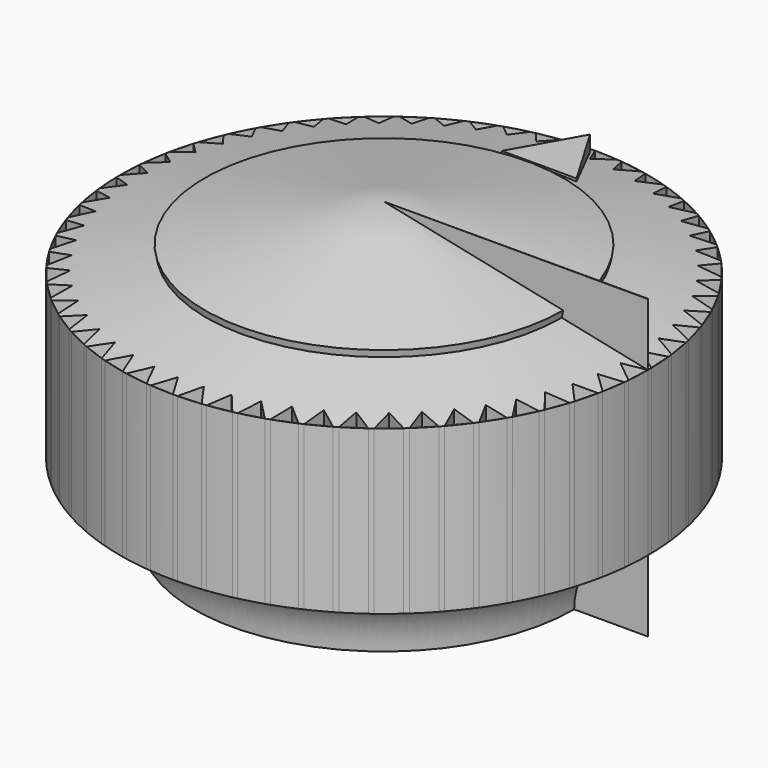
from build123d import *

# Parameters (mm, degrees)
F1_R             = 14.097
F2_DEPTH         = 15.875
F4_ANGLE         = 359.9
F6_DEPTH         = 0.635
F7_DEPTH         = 8.3566
F9_DEPTH         = 11.43
F11_DEPTH        = 15.876
F11_COPIES_COUNT = 60


# Not quite as in the source:
# - a pattern or mirror of a feature is missing from the dataset's text; its kind, count and spacing are read off the source's solid


with BuildPart() as f2:
    # F1 (on Top) → F2 (new body)
    with BuildSketch(Plane.XY):
        Circle(F1_R)
    extrude(amount=F2_DEPTH)

    # F3 (on Front) → F4 (revolve, cut)
    with BuildSketch(Plane.XZ):
        Polygon((14.5759196816, 15.875), (0, 15.875), (9.5739045491, 13.8729814857), (9.4959196816, 13.5000480326), (14.4887969726, 12.4559773794), (14.5759196816, 12.827), align=None)
        with BuildLine():
            Line((14.097, 0), (14.097, 3.8218105259))
            ThreePointArc((14.097, 3.8218105259), (11.3203081245, 2.7434560638), (10.16, 0))
            Line((10.16, 0), (14.097, 0))
        make_face()
    revolve(axis=Axis((0, 0, 15.875), (0, 0, -1)), revolution_arc=F4_ANGLE, mode=Mode.SUBTRACT)

    # F8 (on face) → F9 (cut)
    with BuildSketch(Plane(origin=(0, 0, 0), x_dir=(1, 0, 0), z_dir=(0, 0, -1))):
        with BuildLine():
            Line((-2.2079380086, -2.54), (2.2079380086, -2.54))
            ThreePointArc((2.2079380086, -2.54), (0, 3.3655), (-2.2079380086, -2.54))
        make_face()
    extrude(amount=-F9_DEPTH, mode=Mode.SUBTRACT)

    # F10 (on Top) → F11 (cut, through all)
    with BuildSketch(Plane.XY):
        Polygon((-14.043356659, 1.2286345055), (-14.097, 0), (-13.0711868405, 0.5481573753), align=None)
    f11 = extrude(amount=F11_DEPTH, mode=Mode.SUBTRACT)

    # F11_copies: F11 ×60 about axis
    f11_copies_axis = Axis((0, 0, 0), (0, 0, 1))
    for i in range(1, F11_COPIES_COUNT):
        add(f11.rotate(f11_copies_axis, i * 360 / F11_COPIES_COUNT), mode=Mode.SUBTRACT)


with BuildPart() as f6:
    # F5 (on offset) → F6 (new body)
    with BuildSketch(Plane.XY.offset(5.08)):
        Polygon((2.0429782829, 10.304846555), (0, 13.759015128), (-1.9492893441, 10.304846555), align=None)
    extrude(amount=F6_DEPTH)


with BuildPart() as f7:
    # F5 (on offset) → F7 (new body)
    with BuildSketch(Plane.XY.offset(5.08)):
        Polygon((2.0429782829, 10.304846555), (0, 13.759015128), (-1.9492893441, 10.304846555), align=None)
    extrude(amount=F7_DEPTH)


solid = Compound([f2.part, f6.part, f7.part])
